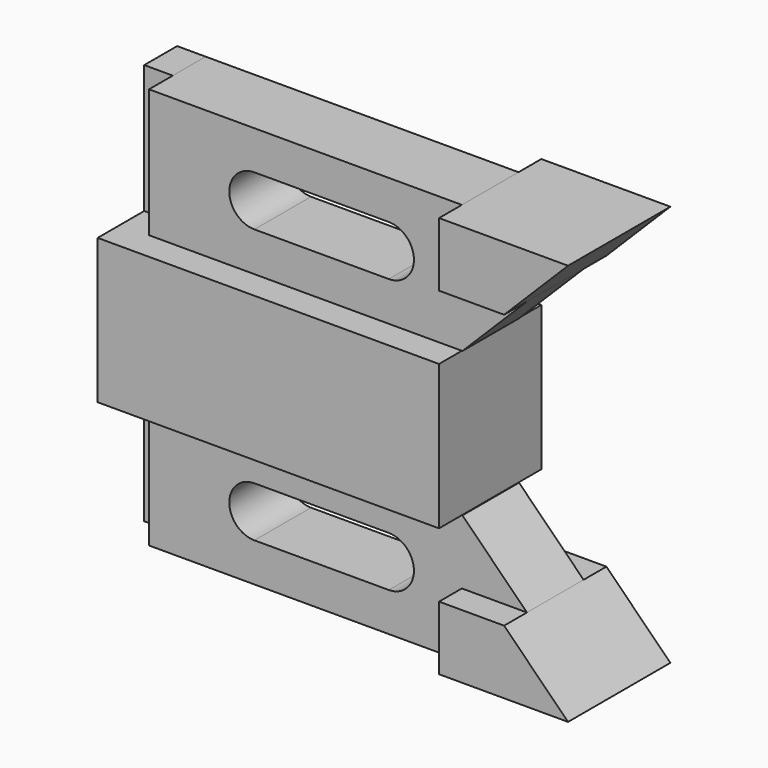
from build123d import *

# Parameters (mm, degrees)
F1_DEPTH  = 7.874
F2_DEPTH  = 14.224
F0_W      = 6.35
F0_H      = 16.0956901618
F0_W_2    = 69.596
F3_DEPTH  = 7.874
F3_FACE_W = 6.35
F3_FACE_H = 28.575
F4_DEPTH  = 6.604


with BuildPart() as f1:
    # F0 (on Front) → F1 (new body, symmetric)
    with BuildSketch(Plane.XZ):
        Polygon((38.6365454535, 5.5099498674), (-30.9594545465, 5.5099498674), (-30.9594545465, -23.0650501326), (38.6365454535, -23.0650501326), (38.6365454535, -8.8410501326), (53.1145454535, -8.8410501326), (38.7635454535, 5.5099498674), align=None)
        with BuildLine():
            ThreePointArc((-13.1061429274, -8.8410501326), (-11.4694556207, -4.8897374393), (-7.5181429274, -3.2530501326))
            Line((-7.5181429274, -3.2530501326), (22.3805454535, -3.2530501326))
            ThreePointArc((22.3805454535, -3.2530501326), (27.9685454535, -8.8410501326), (22.3805454535, -14.4290501326))
            Line((22.3805454535, -14.4290501326), (-7.5181429274, -14.4290501326))
            ThreePointArc((-7.5181429274, -14.4290501326), (-11.4694556207, -12.7923628258), (-13.1061429274, -8.8410501326))
        make_face(mode=Mode.SUBTRACT)
    extrude(amount=F1_DEPTH, both=True)


with BuildPart() as f1b:
    # F0 (on Front) → F1, piece 2 (new body, symmetric)
    with BuildSketch(Plane.XZ):
        Polygon((38.6365454535, 66.276330191), (-30.9594545465, 66.276330191), (-30.9594545465, 37.701330191), (38.6365454535, 37.701330191), (38.7635454535, 37.701330191), (53.1145454535, 52.052330191), (38.6365454535, 52.052330191), align=None)
        with BuildLine():
            Line((22.3805454535, 46.464330191), (-7.5181429274, 46.464330191))
            ThreePointArc((-7.5181429274, 46.464330191), (-11.4694556207, 48.1010174977), (-13.1061429274, 52.052330191))
            ThreePointArc((-13.1061429274, 52.052330191), (-11.4694556207, 56.0036428842), (-7.5181429274, 57.640330191))
            Line((-7.5181429274, 57.640330191), (22.3805454535, 57.640330191))
            ThreePointArc((22.3805454535, 57.640330191), (27.9685454535, 52.052330191), (22.3805454535, 46.464330191))
        make_face(mode=Mode.SUBTRACT)
    extrude(amount=F1_DEPTH, both=True)


with BuildPart() as f2:
    # F0 (on Front) → F2 (new body, symmetric)
    with BuildSketch(Plane.XZ):
        Polygon((38.6365454535, -8.8410501326), (38.6365454535, -23.0650501326), (67.3385454535, -23.0650501326), (53.1145454535, -8.8410501326), align=None)
    extrude(amount=F2_DEPTH, both=True)


with BuildPart() as f2b:
    # F0 (on Front) → F2, piece 2 (new body, symmetric)
    with BuildSketch(Plane.XZ):
        with Locations((-34.1344545465, 13.5577949483)):
            Rectangle(F0_W, F0_H)
        with Locations((3.8385454535, 13.5577949483)):
            Rectangle(F0_W_2, F0_H)
        with Locations((3.8385454535, 29.6534851101)):
            Rectangle(F0_W_2, F0_H)
        with Locations((-34.1344545465, 29.6534851101)):
            Rectangle(F0_W, F0_H)
    extrude(amount=F2_DEPTH, both=True)


with BuildPart() as f2c:
    # F0 (on Front) → F2, piece 3 (new body, symmetric)
    with BuildSketch(Plane.XZ):
        Polygon((67.3385454535, 66.276330191), (38.6365454535, 66.276330191), (38.6365454535, 52.052330191), (53.1145454535, 52.052330191), align=None)
    extrude(amount=F2_DEPTH, both=True)


with BuildPart() as f3:
    # F0 (on Front) → F3 (new body, symmetric)
    with BuildSketch(Plane.XZ):
        Polygon((-30.9594545465, 66.276330191), (-37.3094545465, 66.276330191), (-37.3094545465, 52.052330191), (-37.3094545465, 37.701330191), (-30.9594545465, 37.701330191), align=None)
    extrude(amount=F3_DEPTH, both=True)


with BuildPart() as f3b:
    # F0 (on Front) → F3, piece 2 (new body, symmetric)
    with BuildSketch(Plane.XZ):
        Polygon((-30.9594545465, -23.0650501326), (-30.9594545465, 5.5099498674), (-37.3094545465, 5.5099498674), (-37.3094545465, -8.8410501326), (-37.3094545465, -23.0650501326), align=None)
    extrude(amount=F3_DEPTH, both=True)


with BuildPart() as f4_tool:
    # F3_face (on face) → F4 (new body)
    with BuildSketch(Plane(origin=(-34.1344545465, -7.874, -8.7775501326), x_dir=(1, 0, 0), z_dir=(0, -1, 0))):
        Rectangle(F3_FACE_W, F3_FACE_H)
        with Locations((0, 60.7663803235)):
            Rectangle(F3_FACE_W, F3_FACE_H)
    extrude(amount=-F4_DEPTH)


with BuildPart() as f3_1:
    add(f3.part)

    # F4: cut by f4_tool
    add(f4_tool.part, mode=Mode.SUBTRACT)


with BuildPart() as f3b_1:
    add(f3b.part)

    # F4: cut by f4_tool
    add(f4_tool.part, mode=Mode.SUBTRACT)


solid = Compound([f1.part, f1b.part, f2.part, f2b.part, f2c.part, f3_1.part, f3b_1.part])
